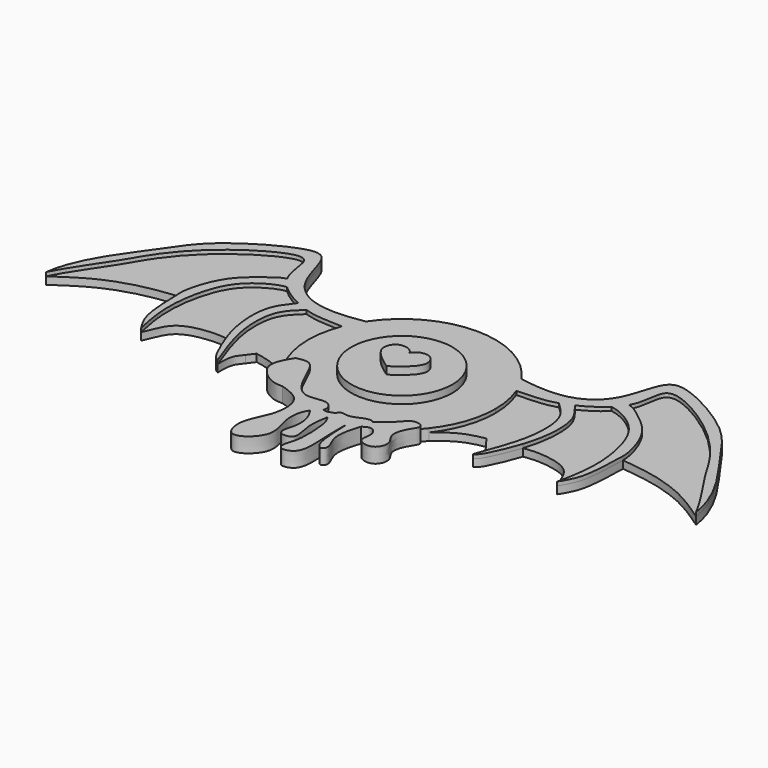
from build123d import *

# Parameters (mm, degrees)
F1_DEPTH = 3
F2_R     = 13.5064277213
F3_DEPTH = 5
F4_DEPTH = 2
F5_DEPTH = 3
F7_DEPTH = 4
F9_DEPTH = 2


with BuildPart() as f1:
    # F0 (on Top) → F1 (new body)
    with BuildSketch(Plane.XY):
        with BuildLine():
            ThreePointArc((-19.6218875172, -15.4913372651), (0, -25), (19.6218875172, -15.4913372651))
            add(Edge.make_bspline(
                [(20.7636337812, 13.92377507), (18.884492427, 12.8973675107), (13.2694896297, 9.830391573), (17.0839746859, -5.3747888898), (19.6218875172, -15.4913372651)],
                knots=[0, 0, 0, 0, 0.3346643665, 1, 1, 1, 1], degree=3))
            ThreePointArc((20.7636337812, 13.92377507), (0, 25), (-20.7636337812, 13.92377507))
            add(Edge.make_bspline(
                [(-20.7636337812, 13.92377507), (-18.884492427, 12.8973675107), (-13.2694896297, 9.830391573), (-17.0839746859, -5.3747888898), (-19.6218875172, -15.4913372651)],
                knots=[0, 0, 0, 0, 0.3346643665, 1, 1, 1, 1], degree=3))
        make_face()
        with BuildLine():
            ThreePointArc((19.6218875172, -15.4913372651), (23.61723087, -8.1991710578), (25, 0))
            ThreePointArc((25, 0), (24.5689951544, 4.6221723357), (23.2908418319, 9.0849703775))
            ThreePointArc((23.2908418319, 9.0849703775), (22.1597092287, 11.5735598197), (20.7636337812, 13.92377507))
            add(Edge.make_bspline(
                [(20.7636337812, 13.92377507), (18.884492427, 12.8973675107), (13.2694896297, 9.830391573), (17.0839746859, -5.3747888898), (19.6218875172, -15.4913372651)],
                knots=[0, 0, 0, 0, 0.3346643665, 1, 1, 1, 1], degree=3))
        make_face()
        with BuildLine():
            ThreePointArc((-23.2908418319, 9.0849703775), (-24.7259844978, -3.6912993126), (-19.6218875172, -15.4913372651))
            add(Edge.make_bspline(
                [(-20.7636337812, 13.92377507), (-18.884492427, 12.8973675107), (-13.2694896297, 9.830391573), (-17.0839746859, -5.3747888898), (-19.6218875172, -15.4913372651)],
                knots=[0, 0, 0, 0, 0.3346643665, 1, 1, 1, 1], degree=3))
            ThreePointArc((-20.7636337812, 13.92377507), (-22.1597092287, 11.5735598197), (-23.2908418319, 9.0849703775))
        make_face()
    extrude(amount=F1_DEPTH)

    # F2 (on Top) → F3 (join)
    with BuildSketch(Plane.XY):
        Circle(F2_R)
    extrude(amount=F3_DEPTH)

    # F0 (on Top) → F4 (join)
    with BuildSketch(Plane.XY):
        with BuildLine():
            ThreePointArc((20.7636337812, 13.92377507), (22.1597092287, 11.5735598197), (23.2908418319, 9.0849703775))
            add(Edge.make_bspline(
                [(23.2908418319, 9.0849703775), (27.8215143515, 9.3257680742), (30.2320226011, 9.1590800923), (33.7177366018, 10.2821364999)],
                knots=[0, 0, 0, 0, 0.1231403921, 0.1231403921, 0.1231403921, 0.1231403921], degree=3))
            add(Edge.make_bspline(
                [(33.7177366018, 10.2821364999), (34.7454077104, 10.6132401484), (35.866536795, 11.0564496893), (37.004531993, 11.5978625395)],
                knots=[0.1231403921, 0.1231403921, 0.1231403921, 0.1231403921, 0.1594450984, 0.1594450984, 0.1594450984, 0.1594450984], degree=3))
            add(Edge.make_bspline(
                [(37.004531993, 11.5978625395), (39.2474500295, 12.6649537267), (41.555886116, 14.1135251746), (43.3434300018, 15.8371345407)],
                knots=[0.1594450984, 0.1594450984, 0.1594450984, 0.1594450984, 0.2309994255, 0.2309994255, 0.2309994255, 0.2309994255], degree=3))
            add(Edge.make_bspline(
                [(43.3434300018, 15.8371345407), (44.2810928585, 16.7412603051), (45.0754287668, 17.7210645793), (45.641798526, 18.7611840665)],
                knots=[0.2309994255, 0.2309994255, 0.2309994255, 0.2309994255, 0.2685335165, 0.2685335165, 0.2685335165, 0.2685335165], degree=3))
            add(Edge.make_bspline(
                [(45.641798526, 18.7611840665), (47.3352689159, 21.8711868955), (46.777744727, 27.7747473366), (51.8560066338, 29.065553317), (66.3600577374, 20.2512677808), (74.7298542288, 9.6960609054), (77.7930462557, 3.5527051654), (84.7415977894, -6.1442317778), (86.8003591895, -10.2821364999)],
                knots=[0.2685335165, 0.2685335165, 0.2685335165, 0.2685335165, 0.3807620926, 0.4500912377, 0.6051903106, 0.7450551623, 0.8470726585, 1, 1, 1, 1], degree=3))
            add(Edge.make_bspline(
                [(20.7636337812, 13.92377507), (25.353260156, 13.083604301), (34.3722799665, 12.4739559617), (43.1666874947, 19.3658325346), (44.7883389447, 31.8865702273), (51.6235191398, 32.3410311281), (68.757647719, 22.5890249267), (75.2339965242, 11.4273433149), (85.5971213344, -1.5157287213), (86.8003591895, -10.2821364999)],
                knots=[0, 0, 0, 0, 0.1438051462, 0.2702269745, 0.4006587664, 0.4888335416, 0.6586500337, 0.8053535671, 1, 1, 1, 1], degree=3))
        make_face()
        with BuildLine():
            ThreePointArc((19.6218875172, -15.4913372651), (23.61723087, -8.1991710578), (25, 0))
            ThreePointArc((25, 0), (24.5689951544, 4.6221723357), (23.2908418319, 9.0849703775))
            ThreePointArc((23.2908418319, 9.0849703775), (22.1597092287, 11.5735598197), (20.7636337812, 13.92377507))
            add(Edge.make_bspline(
                [(20.7636337812, 13.92377507), (18.884492427, 12.8973675107), (13.2694896297, 9.830391573), (17.0839746859, -5.3747888898), (19.6218875172, -15.4913372651)],
                knots=[0, 0, 0, 0, 0.3346643665, 1, 1, 1, 1], degree=3))
        make_face()
        with BuildLine():
            ThreePointArc((23.2908418319, 9.0849703775), (24.5689951544, 4.6221723357), (25, 0))
            ThreePointArc((25, 0), (23.61723087, -8.1991710578), (19.6218875172, -15.4913372651))
            add(Edge.make_bspline(
                [(19.6218875172, -15.4913372651), (21.4152102231, -14.0609489213), (24.8604058768, -11.2746200768), (28.7928801922, -10.5001506768), (30.6888949126, -10.1227229461)],
                knots=[0, 0, 0, 0, 0.5172233423, 1, 1, 1, 1], degree=3))
            add(Edge.make_bspline(
                [(32.1116161516, -12.0142660523), (31.6373757386, -11.3837516835), (31.1631353256, -10.7532373148), (30.6888949126, -10.1227229461)],
                knots=[0, 0, 0, 0, 2.3668694612, 2.3668694612, 2.3668694612, 2.3668694612], degree=3))
            add(Edge.make_bspline(
                [(32.1116161516, -12.0142660523), (32.776720922, -12.8822985255), (34.1447409362, -14.3321949992), (34.1047637318, -17.2769145921), (34.0780636316, -18.8904348761)],
                knots=[0, 0, 0, 0, 0.4499025437, 1, 1, 1, 1], degree=3))
            add(Edge.make_bspline(
                [(33.7177366018, 10.2821364999), (35.3645415529, 8.7757476619), (38.884943387, 5.4848056386), (38.8140830901, -4.1284440887), (37.0736184249, -10.5819579136), (35.282158389, -15.8523198225), (34.0780636316, -18.8904348761)],
                knots=[0, 0, 0, 0, 0.2318500383, 0.4998701646, 0.7334854658, 1, 1, 1, 1], degree=3))
            add(Edge.make_bspline(
                [(23.2908418319, 9.0849703775), (27.8215143515, 9.3257680742), (30.2320226011, 9.1590800923), (33.7177366018, 10.2821364999)],
                knots=[0, 0, 0, 0, 0.1231403921, 0.1231403921, 0.1231403921, 0.1231403921], degree=3))
        make_face()
        with BuildLine():
            add(Edge.make_bspline(
                [(33.7177366018, 10.2821364999), (34.7454077104, 10.6132401484), (35.866536795, 11.0564496893), (37.004531993, 11.5978625395)],
                knots=[0.1231403921, 0.1231403921, 0.1231403921, 0.1231403921, 0.1594450984, 0.1594450984, 0.1594450984, 0.1594450984], degree=3))
            add(Edge.make_bspline(
                [(33.7177366018, 10.2821364999), (35.3645415529, 8.7757476619), (38.884943387, 5.4848056386), (38.8140830901, -4.1284440887), (37.0736184249, -10.5819579136), (35.282158389, -15.8523198225), (34.0780636316, -18.8904348761)],
                knots=[0, 0, 0, 0, 0.2318500383, 0.4998701646, 0.7334854658, 1, 1, 1, 1], degree=3))
            add(Edge.make_bspline(
                [(39.3599004471, -8.7854920866), (38.7249404903, -10.7452749087), (37.0180617267, -14.9012626381), (35.2493275964, -18.5335928874), (34.0780636316, -18.8904348761)],
                knots=[0.6277129418, 0.6277129418, 0.6277129418, 0.6277129418, 0.792816444, 1, 1, 1, 1], degree=3))
            add(Edge.make_bspline(
                [(37.004531993, 11.5978625395), (38.0800679502, 10.0046793736), (41.3336069296, 6.7268291074), (41.1834657071, -2.2502985215), (39.8295408824, -7.3359624778), (39.3599004471, -8.7854920866)],
                knots=[0, 0, 0, 0, 0.2173363693, 0.5055961378, 0.6277129418, 0.6277129418, 0.6277129418, 0.6277129418], degree=3))
        make_face()
        with BuildLine():
            add(Edge.make_bspline(
                [(37.004531993, 11.5978625395), (39.2474500295, 12.6649537267), (41.555886116, 14.1135251746), (43.3434300018, 15.8371345407)],
                knots=[0.1594450984, 0.1594450984, 0.1594450984, 0.1594450984, 0.2309994255, 0.2309994255, 0.2309994255, 0.2309994255], degree=3))
            add(Edge.make_bspline(
                [(37.004531993, 11.5978625395), (38.0800679502, 10.0046793736), (41.3336069296, 6.7268291074), (41.1834657071, -2.2502985215), (39.8295408824, -7.3359624778), (39.3599004471, -8.7854920866)],
                knots=[0, 0, 0, 0, 0.2173363693, 0.5055961378, 0.6277129418, 0.6277129418, 0.6277129418, 0.6277129418], degree=3))
            add(Edge.make_bspline(
                [(55.5573105812, -17.6151320338), (54.4439075888, -14.9875635555), (52.9703835571, -10.411043477), (46.6717355198, -8.6507292972), (42.2245726074, -8.3797506367), (40.2332096515, -8.6600986878), (39.3599004471, -8.7854920866)],
                knots=[0, 0, 0, 0, 0.3047383368, 0.5764576192, 0.8133522424, 1, 1, 1, 1], degree=3))
            add(Edge.make_bspline(
                [(43.3434300018, 15.8371345407), (45.3565623966, 15.5676262825), (49.9854795603, 13.2408710445), (54.5376514308, 8.1613285539), (57.1013516863, -1.3778788699), (57.1238501467, -10.2186225385), (56.0702038202, -15.2273425566), (55.5573105812, -17.6151320338)],
                knots=[0, 0, 0, 0, 0.1860076727, 0.3714288806, 0.5926344587, 0.8055769314, 1, 1, 1, 1], degree=3))
        make_face()
        with BuildLine():
            add(Edge.make_bspline(
                [(45.641798526, 18.7611840665), (47.0236524725, 18.4958354205), (50.5733406235, 15.7663353525), (56.3104736797, 11.1079119823), (58.8622688049, 3.2726876511), (59.0809752339, 0.6245344364), (59.0938226065, 0)],
                knots=[0, 0, 0, 0, 0.146943127, 0.3231645985, 0.5131967694, 0.5724247553, 0.5724247553, 0.5724247553, 0.5724247553], degree=3))
            add(Edge.make_bspline(
                [(43.3434300018, 15.8371345407), (44.2810928585, 16.7412603051), (45.0754287668, 17.7210645793), (45.641798526, 18.7611840665)],
                knots=[0.2309994255, 0.2309994255, 0.2309994255, 0.2309994255, 0.2685335165, 0.2685335165, 0.2685335165, 0.2685335165], degree=3))
            add(Edge.make_bspline(
                [(43.3434300018, 15.8371345407), (45.3565623966, 15.5676262825), (49.9854795603, 13.2408710445), (54.5376514308, 8.1613285539), (57.1013516863, -1.3778788699), (57.1238501467, -10.2186225385), (56.0702038202, -15.2273425566), (55.5573105812, -17.6151320338)],
                knots=[0, 0, 0, 0, 0.1860076727, 0.3714288806, 0.5926344587, 0.8055769314, 1, 1, 1, 1], degree=3))
            add(Edge.make_bspline(
                [(59.0938226065, 0), (59.1104927586, -0.8103667818), (58.9358631638, -3.6588287886), (58.782367202, -12.4944121501), (56.5431938855, -16.0569735079), (55.5573105812, -17.6151320338)],
                knots=[0.5724247553, 0.5724247553, 0.5724247553, 0.5724247553, 0.6492762299, 0.8452276156, 1, 1, 1, 1], degree=3))
        make_face()
        with BuildLine():
            add(Edge.make_bspline(
                [(59.0938226065, 0), (62.0265888913, -0.341290779), (68.0943487487, -1.0474058551), (78.0033682979, -4.2880779786), (83.850491985, -8.272167765), (86.8003591895, -10.2821364999)],
                knots=[0, 0, 0, 0, 0.3167243267, 0.6552882052, 1, 1, 1, 1], degree=3))
            add(Edge.make_bspline(
                [(45.641798526, 18.7611840665), (47.3352689159, 21.8711868955), (46.777744727, 27.7747473366), (51.8560066338, 29.065553317), (66.3600577374, 20.2512677808), (74.7298542288, 9.6960609054), (77.7930462557, 3.5527051654), (84.7415977894, -6.1442317778), (86.8003591895, -10.2821364999)],
                knots=[0.2685335165, 0.2685335165, 0.2685335165, 0.2685335165, 0.3807620926, 0.4500912377, 0.6051903106, 0.7450551623, 0.8470726585, 1, 1, 1, 1], degree=3))
            add(Edge.make_bspline(
                [(45.641798526, 18.7611840665), (47.0236524725, 18.4958354205), (50.5733406235, 15.7663353525), (56.3104736797, 11.1079119823), (58.8622688049, 3.2726876511), (59.0809752339, 0.6245344364), (59.0938226065, 0)],
                knots=[0, 0, 0, 0, 0.146943127, 0.3231645985, 0.5131967694, 0.5724247553, 0.5724247553, 0.5724247553, 0.5724247553], degree=3))
        make_face()
        with BuildLine():
            add(Edge.make_bspline(
                [(-19.6218875172, -15.4913372651), (-21.4152102231, -14.0609489213), (-24.8604058768, -11.2746200768), (-28.7928801922, -10.5001506768), (-30.6888949126, -10.1227229461)],
                knots=[0, 0, 0, 0, 0.5172233423, 1, 1, 1, 1], degree=3))
            ThreePointArc((-19.6218875172, -15.4913372651), (-24.7259844978, -3.6912993126), (-23.2908418319, 9.0849703775))
            add(Edge.make_bspline(
                [(-23.2908418319, 9.0849703775), (-27.8215143515, 9.3257680742), (-30.2320226011, 9.1590800923), (-33.7177366018, 10.2821364999)],
                knots=[0, 0, 0, 0, 0.1231403921, 0.1231403921, 0.1231403921, 0.1231403921], degree=3))
            add(Edge.make_bspline(
                [(-33.7177366018, 10.2821364999), (-35.3645415529, 8.7757476619), (-38.884943387, 5.4848056386), (-38.8140830901, -4.1284440887), (-37.0736184249, -10.5819579136), (-35.282158389, -15.8523198225), (-34.0780636316, -18.8904348761)],
                knots=[0, 0, 0, 0, 0.2318500383, 0.4998701646, 0.7334854658, 1, 1, 1, 1], degree=3))
            add(Edge.make_bspline(
                [(-32.1116161516, -12.0142660523), (-32.776720922, -12.8822985255), (-34.1447409362, -14.3321949992), (-34.1047637318, -17.2769145921), (-34.0780636316, -18.8904348761)],
                knots=[0, 0, 0, 0, 0.4499025437, 1, 1, 1, 1], degree=3))
            add(Edge.make_bspline(
                [(-32.1116161516, -12.0142660523), (-31.6373757386, -11.3837516835), (-31.1631353256, -10.7532373148), (-30.6888949126, -10.1227229461)],
                knots=[0, 0, 0, 0, 2.3668694612, 2.3668694612, 2.3668694612, 2.3668694612], degree=3))
        make_face()
        with BuildLine():
            add(Edge.make_bspline(
                [(-37.004531993, 11.5978625395), (-38.0800679502, 10.0046793736), (-41.3336069296, 6.7268291074), (-41.1834657071, -2.2502985215), (-39.8295408824, -7.3359624778), (-39.3599004471, -8.7854920866)],
                knots=[0, 0, 0, 0, 0.2173363693, 0.5055961378, 0.6277129418, 0.6277129418, 0.6277129418, 0.6277129418], degree=3))
            add(Edge.make_bspline(
                [(-37.004531993, 11.5978625395), (-39.2474500295, 12.6649537267), (-41.555886116, 14.1135251746), (-43.3434300018, 15.8371345407)],
                knots=[0.1594450984, 0.1594450984, 0.1594450984, 0.1594450984, 0.2309994255, 0.2309994255, 0.2309994255, 0.2309994255], degree=3))
            add(Edge.make_bspline(
                [(-43.3434300018, 15.8371345407), (-45.3565623966, 15.5676262825), (-49.9854795603, 13.2408710445), (-54.5376514308, 8.1613285539), (-57.1013516863, -1.3778788699), (-57.1238501467, -10.2186225385), (-56.0702038202, -15.2273425566), (-55.5573105812, -17.6151320338)],
                knots=[0, 0, 0, 0, 0.1860076727, 0.3714288806, 0.5926344587, 0.8055769314, 1, 1, 1, 1], degree=3))
            add(Edge.make_bspline(
                [(-55.5573105812, -17.6151320338), (-54.4439075888, -14.9875635555), (-52.9703835571, -10.411043477), (-46.6717355198, -8.6507292972), (-42.2245726074, -8.3797506367), (-40.2332096515, -8.6600986878), (-39.3599004471, -8.7854920866)],
                knots=[0, 0, 0, 0, 0.3047383368, 0.5764576192, 0.8133522424, 1, 1, 1, 1], degree=3))
        make_face()
        with BuildLine():
            add(Edge.make_bspline(
                [(-33.7177366018, 10.2821364999), (-35.3645415529, 8.7757476619), (-38.884943387, 5.4848056386), (-38.8140830901, -4.1284440887), (-37.0736184249, -10.5819579136), (-35.282158389, -15.8523198225), (-34.0780636316, -18.8904348761)],
                knots=[0, 0, 0, 0, 0.2318500383, 0.4998701646, 0.7334854658, 1, 1, 1, 1], degree=3))
            add(Edge.make_bspline(
                [(-33.7177366018, 10.2821364999), (-34.7454077104, 10.6132401484), (-35.866536795, 11.0564496893), (-37.004531993, 11.5978625395)],
                knots=[0.1231403921, 0.1231403921, 0.1231403921, 0.1231403921, 0.1594450984, 0.1594450984, 0.1594450984, 0.1594450984], degree=3))
            add(Edge.make_bspline(
                [(-37.004531993, 11.5978625395), (-38.0800679502, 10.0046793736), (-41.3336069296, 6.7268291074), (-41.1834657071, -2.2502985215), (-39.8295408824, -7.3359624778), (-39.3599004471, -8.7854920866)],
                knots=[0, 0, 0, 0, 0.2173363693, 0.5055961378, 0.6277129418, 0.6277129418, 0.6277129418, 0.6277129418], degree=3))
            add(Edge.make_bspline(
                [(-39.3599004471, -8.7854920866), (-38.7249404903, -10.7452749087), (-37.0180617267, -14.9012626381), (-35.2493275964, -18.5335928874), (-34.0780636316, -18.8904348761)],
                knots=[0.6277129418, 0.6277129418, 0.6277129418, 0.6277129418, 0.792816444, 1, 1, 1, 1], degree=3))
        make_face()
        with BuildLine():
            ThreePointArc((-23.2908418319, 9.0849703775), (-22.1597092287, 11.5735598197), (-20.7636337812, 13.92377507))
            add(Edge.make_bspline(
                [(-20.7636337812, 13.92377507), (-25.353260156, 13.083604301), (-34.3722799665, 12.4739559617), (-43.1666874947, 19.3658325346), (-44.7883389447, 31.8865702273), (-51.6235191398, 32.3410311281), (-68.757647719, 22.5890249267), (-75.2339965242, 11.4273433149), (-85.5971213344, -1.5157287213), (-86.8003591895, -10.2821364999)],
                knots=[0, 0, 0, 0, 0.1438051462, 0.2702269745, 0.4006587664, 0.4888335416, 0.6586500337, 0.8053535671, 1, 1, 1, 1], degree=3))
            add(Edge.make_bspline(
                [(-45.641798526, 18.7611840665), (-47.3352689159, 21.8711868955), (-46.777744727, 27.7747473366), (-51.8560066338, 29.065553317), (-66.3600577374, 20.2512677808), (-74.7298542288, 9.6960609054), (-77.7930462557, 3.5527051654), (-84.7415977894, -6.1442317778), (-86.8003591895, -10.2821364999)],
                knots=[0.2685335165, 0.2685335165, 0.2685335165, 0.2685335165, 0.3807620926, 0.4500912377, 0.6051903106, 0.7450551623, 0.8470726585, 1, 1, 1, 1], degree=3))
            add(Edge.make_bspline(
                [(-43.3434300018, 15.8371345407), (-44.2810928585, 16.7412603051), (-45.0754287668, 17.7210645793), (-45.641798526, 18.7611840665)],
                knots=[0.2309994255, 0.2309994255, 0.2309994255, 0.2309994255, 0.2685335165, 0.2685335165, 0.2685335165, 0.2685335165], degree=3))
            add(Edge.make_bspline(
                [(-37.004531993, 11.5978625395), (-39.2474500295, 12.6649537267), (-41.555886116, 14.1135251746), (-43.3434300018, 15.8371345407)],
                knots=[0.1594450984, 0.1594450984, 0.1594450984, 0.1594450984, 0.2309994255, 0.2309994255, 0.2309994255, 0.2309994255], degree=3))
            add(Edge.make_bspline(
                [(-33.7177366018, 10.2821364999), (-34.7454077104, 10.6132401484), (-35.866536795, 11.0564496893), (-37.004531993, 11.5978625395)],
                knots=[0.1231403921, 0.1231403921, 0.1231403921, 0.1231403921, 0.1594450984, 0.1594450984, 0.1594450984, 0.1594450984], degree=3))
            add(Edge.make_bspline(
                [(-23.2908418319, 9.0849703775), (-27.8215143515, 9.3257680742), (-30.2320226011, 9.1590800923), (-33.7177366018, 10.2821364999)],
                knots=[0, 0, 0, 0, 0.1231403921, 0.1231403921, 0.1231403921, 0.1231403921], degree=3))
        make_face()
        with BuildLine():
            add(Edge.make_bspline(
                [(-45.641798526, 18.7611840665), (-47.3352689159, 21.8711868955), (-46.777744727, 27.7747473366), (-51.8560066338, 29.065553317), (-66.3600577374, 20.2512677808), (-74.7298542288, 9.6960609054), (-77.7930462557, 3.5527051654), (-84.7415977894, -6.1442317778), (-86.8003591895, -10.2821364999)],
                knots=[0.2685335165, 0.2685335165, 0.2685335165, 0.2685335165, 0.3807620926, 0.4500912377, 0.6051903106, 0.7450551623, 0.8470726585, 1, 1, 1, 1], degree=3))
            add(Edge.make_bspline(
                [(-59.0938226065, 0), (-62.0265888913, -0.341290779), (-68.0943487487, -1.0474058551), (-78.0033682979, -4.2880779786), (-83.850491985, -8.272167765), (-86.8003591895, -10.2821364999)],
                knots=[0, 0, 0, 0, 0.3167243267, 0.6552882052, 1, 1, 1, 1], degree=3))
            add(Edge.make_bspline(
                [(-45.641798526, 18.7611840665), (-47.0236524725, 18.4958354205), (-50.5733406235, 15.7663353525), (-56.3104736797, 11.1079119823), (-58.8622688049, 3.2726876511), (-59.0809752339, 0.6245344364), (-59.0938226065, 0)],
                knots=[0, 0, 0, 0, 0.146943127, 0.3231645985, 0.5131967694, 0.5724247553, 0.5724247553, 0.5724247553, 0.5724247553], degree=3))
        make_face()
        with BuildLine():
            add(Edge.make_bspline(
                [(-43.3434300018, 15.8371345407), (-44.2810928585, 16.7412603051), (-45.0754287668, 17.7210645793), (-45.641798526, 18.7611840665)],
                knots=[0.2309994255, 0.2309994255, 0.2309994255, 0.2309994255, 0.2685335165, 0.2685335165, 0.2685335165, 0.2685335165], degree=3))
            add(Edge.make_bspline(
                [(-45.641798526, 18.7611840665), (-47.0236524725, 18.4958354205), (-50.5733406235, 15.7663353525), (-56.3104736797, 11.1079119823), (-58.8622688049, 3.2726876511), (-59.0809752339, 0.6245344364), (-59.0938226065, 0)],
                knots=[0, 0, 0, 0, 0.146943127, 0.3231645985, 0.5131967694, 0.5724247553, 0.5724247553, 0.5724247553, 0.5724247553], degree=3))
            add(Edge.make_bspline(
                [(-59.0938226065, 0), (-59.1104927586, -0.8103667818), (-58.9358631638, -3.6588287886), (-58.782367202, -12.4944121501), (-56.5431938855, -16.0569735079), (-55.5573105812, -17.6151320338)],
                knots=[0.5724247553, 0.5724247553, 0.5724247553, 0.5724247553, 0.6492762299, 0.8452276156, 1, 1, 1, 1], degree=3))
            add(Edge.make_bspline(
                [(-43.3434300018, 15.8371345407), (-45.3565623966, 15.5676262825), (-49.9854795603, 13.2408710445), (-54.5376514308, 8.1613285539), (-57.1013516863, -1.3778788699), (-57.1238501467, -10.2186225385), (-56.0702038202, -15.2273425566), (-55.5573105812, -17.6151320338)],
                knots=[0, 0, 0, 0, 0.1860076727, 0.3714288806, 0.5926344587, 0.8055769314, 1, 1, 1, 1], degree=3))
        make_face()
        with BuildLine():
            ThreePointArc((-23.2908418319, 9.0849703775), (-24.7259844978, -3.6912993126), (-19.6218875172, -15.4913372651))
            add(Edge.make_bspline(
                [(-20.7636337812, 13.92377507), (-18.884492427, 12.8973675107), (-13.2694896297, 9.830391573), (-17.0839746859, -5.3747888898), (-19.6218875172, -15.4913372651)],
                knots=[0, 0, 0, 0, 0.3346643665, 1, 1, 1, 1], degree=3))
            ThreePointArc((-20.7636337812, 13.92377507), (-22.1597092287, 11.5735598197), (-23.2908418319, 9.0849703775))
        make_face()
    extrude(amount=F4_DEPTH)

    # F0 (on Top) → F5 (join)
    with BuildSketch(Plane.XY):
        with BuildLine():
            ThreePointArc((20.7636337812, 13.92377507), (22.1597092287, 11.5735598197), (23.2908418319, 9.0849703775))
            add(Edge.make_bspline(
                [(23.2908418319, 9.0849703775), (27.8215143515, 9.3257680742), (30.2320226011, 9.1590800923), (33.7177366018, 10.2821364999)],
                knots=[0, 0, 0, 0, 0.1231403921, 0.1231403921, 0.1231403921, 0.1231403921], degree=3))
            add(Edge.make_bspline(
                [(33.7177366018, 10.2821364999), (34.7454077104, 10.6132401484), (35.866536795, 11.0564496893), (37.004531993, 11.5978625395)],
                knots=[0.1231403921, 0.1231403921, 0.1231403921, 0.1231403921, 0.1594450984, 0.1594450984, 0.1594450984, 0.1594450984], degree=3))
            add(Edge.make_bspline(
                [(37.004531993, 11.5978625395), (39.2474500295, 12.6649537267), (41.555886116, 14.1135251746), (43.3434300018, 15.8371345407)],
                knots=[0.1594450984, 0.1594450984, 0.1594450984, 0.1594450984, 0.2309994255, 0.2309994255, 0.2309994255, 0.2309994255], degree=3))
            add(Edge.make_bspline(
                [(43.3434300018, 15.8371345407), (44.2810928585, 16.7412603051), (45.0754287668, 17.7210645793), (45.641798526, 18.7611840665)],
                knots=[0.2309994255, 0.2309994255, 0.2309994255, 0.2309994255, 0.2685335165, 0.2685335165, 0.2685335165, 0.2685335165], degree=3))
            add(Edge.make_bspline(
                [(45.641798526, 18.7611840665), (47.3352689159, 21.8711868955), (46.777744727, 27.7747473366), (51.8560066338, 29.065553317), (66.3600577374, 20.2512677808), (74.7298542288, 9.6960609054), (77.7930462557, 3.5527051654), (84.7415977894, -6.1442317778), (86.8003591895, -10.2821364999)],
                knots=[0.2685335165, 0.2685335165, 0.2685335165, 0.2685335165, 0.3807620926, 0.4500912377, 0.6051903106, 0.7450551623, 0.8470726585, 1, 1, 1, 1], degree=3))
            add(Edge.make_bspline(
                [(20.7636337812, 13.92377507), (25.353260156, 13.083604301), (34.3722799665, 12.4739559617), (43.1666874947, 19.3658325346), (44.7883389447, 31.8865702273), (51.6235191398, 32.3410311281), (68.757647719, 22.5890249267), (75.2339965242, 11.4273433149), (85.5971213344, -1.5157287213), (86.8003591895, -10.2821364999)],
                knots=[0, 0, 0, 0, 0.1438051462, 0.2702269745, 0.4006587664, 0.4888335416, 0.6586500337, 0.8053535671, 1, 1, 1, 1], degree=3))
        make_face()
        with BuildLine():
            add(Edge.make_bspline(
                [(33.7177366018, 10.2821364999), (34.7454077104, 10.6132401484), (35.866536795, 11.0564496893), (37.004531993, 11.5978625395)],
                knots=[0.1231403921, 0.1231403921, 0.1231403921, 0.1231403921, 0.1594450984, 0.1594450984, 0.1594450984, 0.1594450984], degree=3))
            add(Edge.make_bspline(
                [(33.7177366018, 10.2821364999), (35.3645415529, 8.7757476619), (38.884943387, 5.4848056386), (38.8140830901, -4.1284440887), (37.0736184249, -10.5819579136), (35.282158389, -15.8523198225), (34.0780636316, -18.8904348761)],
                knots=[0, 0, 0, 0, 0.2318500383, 0.4998701646, 0.7334854658, 1, 1, 1, 1], degree=3))
            add(Edge.make_bspline(
                [(39.3599004471, -8.7854920866), (38.7249404903, -10.7452749087), (37.0180617267, -14.9012626381), (35.2493275964, -18.5335928874), (34.0780636316, -18.8904348761)],
                knots=[0.6277129418, 0.6277129418, 0.6277129418, 0.6277129418, 0.792816444, 1, 1, 1, 1], degree=3))
            add(Edge.make_bspline(
                [(37.004531993, 11.5978625395), (38.0800679502, 10.0046793736), (41.3336069296, 6.7268291074), (41.1834657071, -2.2502985215), (39.8295408824, -7.3359624778), (39.3599004471, -8.7854920866)],
                knots=[0, 0, 0, 0, 0.2173363693, 0.5055961378, 0.6277129418, 0.6277129418, 0.6277129418, 0.6277129418], degree=3))
        make_face()
        with BuildLine():
            add(Edge.make_bspline(
                [(45.641798526, 18.7611840665), (47.0236524725, 18.4958354205), (50.5733406235, 15.7663353525), (56.3104736797, 11.1079119823), (58.8622688049, 3.2726876511), (59.0809752339, 0.6245344364), (59.0938226065, 0)],
                knots=[0, 0, 0, 0, 0.146943127, 0.3231645985, 0.5131967694, 0.5724247553, 0.5724247553, 0.5724247553, 0.5724247553], degree=3))
            add(Edge.make_bspline(
                [(43.3434300018, 15.8371345407), (44.2810928585, 16.7412603051), (45.0754287668, 17.7210645793), (45.641798526, 18.7611840665)],
                knots=[0.2309994255, 0.2309994255, 0.2309994255, 0.2309994255, 0.2685335165, 0.2685335165, 0.2685335165, 0.2685335165], degree=3))
            add(Edge.make_bspline(
                [(43.3434300018, 15.8371345407), (45.3565623966, 15.5676262825), (49.9854795603, 13.2408710445), (54.5376514308, 8.1613285539), (57.1013516863, -1.3778788699), (57.1238501467, -10.2186225385), (56.0702038202, -15.2273425566), (55.5573105812, -17.6151320338)],
                knots=[0, 0, 0, 0, 0.1860076727, 0.3714288806, 0.5926344587, 0.8055769314, 1, 1, 1, 1], degree=3))
            add(Edge.make_bspline(
                [(59.0938226065, 0), (59.1104927586, -0.8103667818), (58.9358631638, -3.6588287886), (58.782367202, -12.4944121501), (56.5431938855, -16.0569735079), (55.5573105812, -17.6151320338)],
                knots=[0.5724247553, 0.5724247553, 0.5724247553, 0.5724247553, 0.6492762299, 0.8452276156, 1, 1, 1, 1], degree=3))
        make_face()
        with BuildLine():
            ThreePointArc((-23.2908418319, 9.0849703775), (-22.1597092287, 11.5735598197), (-20.7636337812, 13.92377507))
            add(Edge.make_bspline(
                [(-20.7636337812, 13.92377507), (-25.353260156, 13.083604301), (-34.3722799665, 12.4739559617), (-43.1666874947, 19.3658325346), (-44.7883389447, 31.8865702273), (-51.6235191398, 32.3410311281), (-68.757647719, 22.5890249267), (-75.2339965242, 11.4273433149), (-85.5971213344, -1.5157287213), (-86.8003591895, -10.2821364999)],
                knots=[0, 0, 0, 0, 0.1438051462, 0.2702269745, 0.4006587664, 0.4888335416, 0.6586500337, 0.8053535671, 1, 1, 1, 1], degree=3))
            add(Edge.make_bspline(
                [(-45.641798526, 18.7611840665), (-47.3352689159, 21.8711868955), (-46.777744727, 27.7747473366), (-51.8560066338, 29.065553317), (-66.3600577374, 20.2512677808), (-74.7298542288, 9.6960609054), (-77.7930462557, 3.5527051654), (-84.7415977894, -6.1442317778), (-86.8003591895, -10.2821364999)],
                knots=[0.2685335165, 0.2685335165, 0.2685335165, 0.2685335165, 0.3807620926, 0.4500912377, 0.6051903106, 0.7450551623, 0.8470726585, 1, 1, 1, 1], degree=3))
            add(Edge.make_bspline(
                [(-43.3434300018, 15.8371345407), (-44.2810928585, 16.7412603051), (-45.0754287668, 17.7210645793), (-45.641798526, 18.7611840665)],
                knots=[0.2309994255, 0.2309994255, 0.2309994255, 0.2309994255, 0.2685335165, 0.2685335165, 0.2685335165, 0.2685335165], degree=3))
            add(Edge.make_bspline(
                [(-37.004531993, 11.5978625395), (-39.2474500295, 12.6649537267), (-41.555886116, 14.1135251746), (-43.3434300018, 15.8371345407)],
                knots=[0.1594450984, 0.1594450984, 0.1594450984, 0.1594450984, 0.2309994255, 0.2309994255, 0.2309994255, 0.2309994255], degree=3))
            add(Edge.make_bspline(
                [(-33.7177366018, 10.2821364999), (-34.7454077104, 10.6132401484), (-35.866536795, 11.0564496893), (-37.004531993, 11.5978625395)],
                knots=[0.1231403921, 0.1231403921, 0.1231403921, 0.1231403921, 0.1594450984, 0.1594450984, 0.1594450984, 0.1594450984], degree=3))
            add(Edge.make_bspline(
                [(-23.2908418319, 9.0849703775), (-27.8215143515, 9.3257680742), (-30.2320226011, 9.1590800923), (-33.7177366018, 10.2821364999)],
                knots=[0, 0, 0, 0, 0.1231403921, 0.1231403921, 0.1231403921, 0.1231403921], degree=3))
        make_face()
        with BuildLine():
            add(Edge.make_bspline(
                [(-33.7177366018, 10.2821364999), (-35.3645415529, 8.7757476619), (-38.884943387, 5.4848056386), (-38.8140830901, -4.1284440887), (-37.0736184249, -10.5819579136), (-35.282158389, -15.8523198225), (-34.0780636316, -18.8904348761)],
                knots=[0, 0, 0, 0, 0.2318500383, 0.4998701646, 0.7334854658, 1, 1, 1, 1], degree=3))
            add(Edge.make_bspline(
                [(-33.7177366018, 10.2821364999), (-34.7454077104, 10.6132401484), (-35.866536795, 11.0564496893), (-37.004531993, 11.5978625395)],
                knots=[0.1231403921, 0.1231403921, 0.1231403921, 0.1231403921, 0.1594450984, 0.1594450984, 0.1594450984, 0.1594450984], degree=3))
            add(Edge.make_bspline(
                [(-37.004531993, 11.5978625395), (-38.0800679502, 10.0046793736), (-41.3336069296, 6.7268291074), (-41.1834657071, -2.2502985215), (-39.8295408824, -7.3359624778), (-39.3599004471, -8.7854920866)],
                knots=[0, 0, 0, 0, 0.2173363693, 0.5055961378, 0.6277129418, 0.6277129418, 0.6277129418, 0.6277129418], degree=3))
            add(Edge.make_bspline(
                [(-39.3599004471, -8.7854920866), (-38.7249404903, -10.7452749087), (-37.0180617267, -14.9012626381), (-35.2493275964, -18.5335928874), (-34.0780636316, -18.8904348761)],
                knots=[0.6277129418, 0.6277129418, 0.6277129418, 0.6277129418, 0.792816444, 1, 1, 1, 1], degree=3))
        make_face()
        with BuildLine():
            add(Edge.make_bspline(
                [(-43.3434300018, 15.8371345407), (-44.2810928585, 16.7412603051), (-45.0754287668, 17.7210645793), (-45.641798526, 18.7611840665)],
                knots=[0.2309994255, 0.2309994255, 0.2309994255, 0.2309994255, 0.2685335165, 0.2685335165, 0.2685335165, 0.2685335165], degree=3))
            add(Edge.make_bspline(
                [(-45.641798526, 18.7611840665), (-47.0236524725, 18.4958354205), (-50.5733406235, 15.7663353525), (-56.3104736797, 11.1079119823), (-58.8622688049, 3.2726876511), (-59.0809752339, 0.6245344364), (-59.0938226065, 0)],
                knots=[0, 0, 0, 0, 0.146943127, 0.3231645985, 0.5131967694, 0.5724247553, 0.5724247553, 0.5724247553, 0.5724247553], degree=3))
            add(Edge.make_bspline(
                [(-59.0938226065, 0), (-59.1104927586, -0.8103667818), (-58.9358631638, -3.6588287886), (-58.782367202, -12.4944121501), (-56.5431938855, -16.0569735079), (-55.5573105812, -17.6151320338)],
                knots=[0.5724247553, 0.5724247553, 0.5724247553, 0.5724247553, 0.6492762299, 0.8452276156, 1, 1, 1, 1], degree=3))
            add(Edge.make_bspline(
                [(-43.3434300018, 15.8371345407), (-45.3565623966, 15.5676262825), (-49.9854795603, 13.2408710445), (-54.5376514308, 8.1613285539), (-57.1013516863, -1.3778788699), (-57.1238501467, -10.2186225385), (-56.0702038202, -15.2273425566), (-55.5573105812, -17.6151320338)],
                knots=[0, 0, 0, 0, 0.1860076727, 0.3714288806, 0.5926344587, 0.8055769314, 1, 1, 1, 1], degree=3))
        make_face()
    extrude(amount=F5_DEPTH)

    # F6 (on Top) → F7 (join)
    with BuildSketch(Plane.XY):
        with BuildLine():
            add(Edge.make_bspline(
                [(-20.7235760014, -9.6445070811), (-19.40634346, -9.3306596256), (-16.2692731337, -8.5832173173), (-13.8404857628, -15.9262885752), (-9.3698744561, -22.893109603), (-2.8654473112, -19.9783646263), (-1.1182007603, -23.203626034), (-1.5408760969, -24.1634941887), (-1.6355179467, -24.3131122859)],
                knots=[0, 0, 0, 0, 0.0606496106, 0.1444511325, 0.2309256106, 0.3057439584, 0.3606752212, 0.3715110564, 0.3715110564, 0.3715110564, 0.3715110564], degree=3))
            add(Edge.make_bspline(
                [(-20.7235760014, -9.6445070811), (-21.9943953935, -11.7440305486), (-24.535062388, -15.9411575973), (-18.4930641439, -21.2411641402), (-15.918737994, -21.2695682893), (-14.8254489317, -21.2816298766)],
                knots=[0, 0, 0, 0, 0.3654142522, 0.7305034079, 1, 1, 1, 1], degree=3))
            add(Edge.make_bspline(
                [(-3.5070139238, -26.2158849673), (-4.6131211591, -27.5997100414), (-5.6895321201, -32.5921856123), (-1.5713967275, -40.0141150071), (-10.1452453114, -47.029797053), (-12.5639090643, -38.7870466023), (-7.9861304572, -32.4938336445), (-8.0062270704, -23.5381526959), (-12.6120485953, -22.0140884211), (-14.8254489317, -21.2816298766)],
                knots=[0.4169646347, 0.4169646347, 0.4169646347, 0.4169646347, 0.4958206062, 0.5846771067, 0.6693456642, 0.7426699508, 0.8329154656, 0.9197046813, 1, 1, 1, 1], degree=3))
            add(Edge.make_bspline(
                [(-1.6355179467, -24.3131122859), (-2.0325164873, -24.9407222314), (-2.8694397361, -25.418230708), (-3.5070139238, -26.2158849673)],
                knots=[0.3715110564, 0.3715110564, 0.3715110564, 0.3715110564, 0.4169646347, 0.4169646347, 0.4169646347, 0.4169646347], degree=3))
        make_face()
        with BuildLine():
            add(Edge.make_bspline(
                [(1.1985873829, -23.951514107), (0.9671167555, -23.8260086665), (-0.0754281046, -24.5534155095), (-1.0911163539, -24.3982023049), (-1.6355179467, -24.3131122859)],
                knots=[0.8691013178, 0.8691013178, 0.8691013178, 0.8691013178, 0.9301825186, 1, 1, 1, 1], degree=3))
            add(Edge.make_bspline(
                [(-1.6355179467, -24.3131122859), (-2.0325164873, -24.9407222314), (-2.8694397361, -25.418230708), (-3.5070139238, -26.2158849673)],
                knots=[0.3715110564, 0.3715110564, 0.3715110564, 0.3715110564, 0.4169646347, 0.4169646347, 0.4169646347, 0.4169646347], degree=3))
            add(Edge.make_bspline(
                [(-3.5070139238, -26.2158849673), (-2.883400909, -27.2108060416), (-1.5772187189, -29.3053951505), (-1.4367162452, -33.6612041083), (-2.8086719328, -36.8433496475), (-1.5821949157, -38.5187493793), (2.1045932294, -38.0152983382), (0.657934516, -33.3111620091), (0.6247250909, -29.5615780061), (1.0406939075, -27.2379166479), (1.1982494233, -26.2158849673)],
                knots=[0, 0, 0, 0, 0.1031682262, 0.2164685226, 0.3149071194, 0.3837004952, 0.4707341613, 0.580301166, 0.6920239127, 0.7820958486, 0.7820958486, 0.7820958486, 0.7820958486], degree=3))
            add(Edge.make_bspline(
                [(1.1982494233, -26.2158849673), (1.2225125476, -26.0584948459), (1.3705220613, -25.073510707), (1.4757351702, -24.1017861113), (1.1985873829, -23.951514107)],
                knots=[0.7820958486, 0.7820958486, 0.7820958486, 0.7820958486, 0.7959666837, 0.8691013178, 0.8691013178, 0.8691013178, 0.8691013178], degree=3))
        make_face()
        with BuildLine():
            add(Edge.make_bspline(
                [(1.1985873829, -23.951514107), (1.4456187322, -23.5413655037), (2.0607348171, -22.5172449826), (4.569693506, -23.6127308263), (7.6831118026, -21.5738187686), (9.5325944539, -21.6347257364), (9.8100658506, -22.1171975136)],
                knots=[0, 0, 0, 0, 0.0635011481, 0.1450475396, 0.250308378, 0.3247515807, 0.3247515807, 0.3247515807, 0.3247515807], degree=3))
            add(Edge.make_bspline(
                [(1.1982494233, -26.2158849673), (1.2225125476, -26.0584948459), (1.3705220613, -25.073510707), (1.4757351702, -24.1017861113), (1.1985873829, -23.951514107)],
                knots=[0.7820958486, 0.7820958486, 0.7820958486, 0.7820958486, 0.7959666837, 0.8691013178, 0.8691013178, 0.8691013178, 0.8691013178], degree=3))
            add(Edge.make_bspline(
                [(1.1982494233, -26.2158849673), (1.4979284081, -26.7344342174), (2.3511783621, -28.1806505644), (2.8960916753, -32.7060242963), (2.8368634421, -38.6304914955), (1.4698684717, -41.4487670686), (2.0468797086, -43.7835940306), (5.4960568497, -43.0399207048), (6.7358237459, -39.9814740684), (6.4991708276, -34.6131617172), (6.2124354964, -28.3028086529), (6.4117750153, -26.496719569)],
                knots=[0, 0, 0, 0, 0.081756919, 0.2032537912, 0.342202672, 0.4415256683, 0.5150852099, 0.6082203638, 0.7051553265, 0.8401046214, 1, 1, 1, 1], degree=3))
            add(Edge.make_bspline(
                [(9.3381456619, -25.2787085652), (9.196995182, -25.7167954283), (8.3192847319, -28.3791876849), (7.4811663995, -32.8328210461), (10.1657650242, -36.4540025692), (9.0159326644, -38.4196952544), (6.5383496697, -36.8673925358), (6.477853092, -29.0292938872), (6.4117750153, -26.496719569)],
                knots=[0.4130127364, 0.4130127364, 0.4130127364, 0.4130127364, 0.4411392496, 0.5778350075, 0.6865397452, 0.751044758, 0.8255380089, 1, 1, 1, 1], degree=3))
            add(Edge.make_bspline(
                [(9.8100658506, -22.1171975136), (10.1390407634, -22.6892244421), (9.7810766576, -23.9039895378), (9.3381456619, -25.2787085652)],
                knots=[0.3247515807, 0.3247515807, 0.3247515807, 0.3247515807, 0.4130127364, 0.4130127364, 0.4130127364, 0.4130127364], degree=3))
        make_face()
        with BuildLine():
            add(Edge.make_bspline(
                [(9.8100658506, -22.1171975136), (10.9741769979, -21.366557591), (13.3243177082, -19.8511443672), (15.9380704568, -15.7619444396), (19.975953422, -17.2572525302), (17.132914924, -20.4315107657), (16.1901407251, -24.7358698707), (19.1658910663, -27.1540254755), (17.5214979585, -31.8211786857), (11.9489568899, -30.4732240064), (13.8499253148, -26.3691078042), (11.419900129, -23.9422267652), (10.0144666281, -24.8453806809), (9.3381456619, -25.2787085652)],
                knots=[0, 0, 0, 0, 0.1021114388, 0.2061563584, 0.2845912757, 0.3745199668, 0.4749543371, 0.5648277156, 0.6592223078, 0.7554885334, 0.8480624308, 0.9269925885, 1, 1, 1, 1], degree=3))
            add(Edge.make_bspline(
                [(9.8100658506, -22.1171975136), (10.1390407634, -22.6892244421), (9.7810766576, -23.9039895378), (9.3381456619, -25.2787085652)],
                knots=[0.3247515807, 0.3247515807, 0.3247515807, 0.3247515807, 0.4130127364, 0.4130127364, 0.4130127364, 0.4130127364], degree=3))
        make_face()
    extrude(amount=F7_DEPTH)

    # F8 (on face) → F9 (join)
    with BuildSketch(Plane.XY.offset(5)):
        with BuildLine():
            add(Edge.make_bspline(
                [(0, 2.5627594441), (0.3713491606, 3.2004115637), (1.3030946309, 4.1748766312), (4.5424422124, 4.5508958573), (6.7018800161, 0.7320653912), (3.0808820938, -3.0351484952), (1.090913521, -4.3643188649), (0, -5.1289156545)],
                knots=[0, 0, 0, 0, 0.1572489867, 0.341052242, 0.543275427, 0.781305903, 1, 1, 1, 1], degree=3))
            add(Edge.make_bspline(
                [(0, 2.5627594441), (-0.3713491606, 3.2004115637), (-1.3030946309, 4.1748766312), (-4.5424422124, 4.5508958573), (-6.7018800161, 0.7320653912), (-3.0808820938, -3.0351484952), (-1.090913521, -4.3643188649), (0, -5.1289156545)],
                knots=[0, 0, 0, 0, 0.1572489867, 0.341052242, 0.543275427, 0.781305903, 1, 1, 1, 1], degree=3))
        make_face()
    extrude(amount=F9_DEPTH)


solid = f1.part
